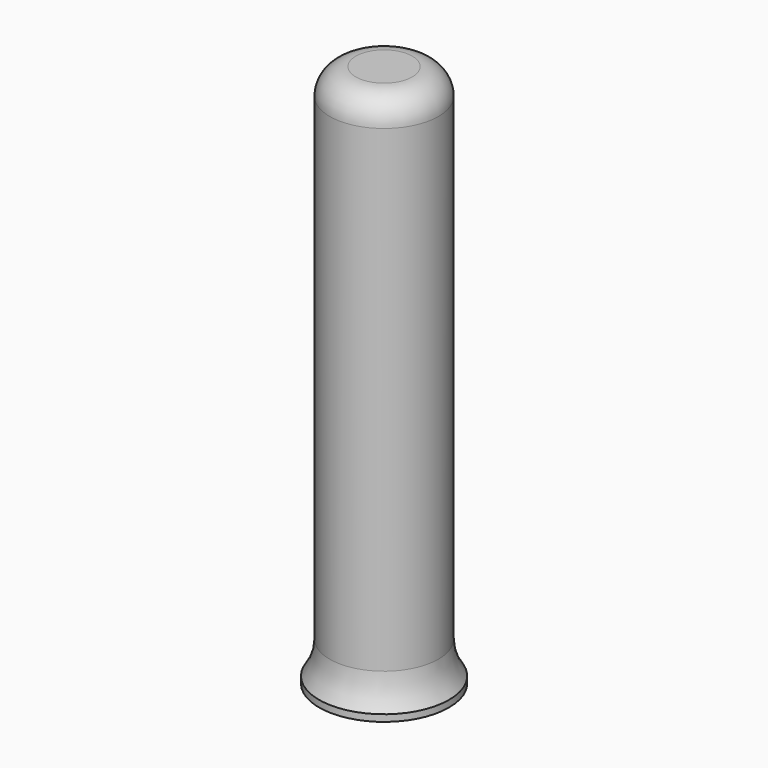
from build123d import *

# Parameters (mm, degrees)
F0_R      = 6.3625068229
F1_DEPTH  = 63.5
F2_R      = 4.7646286231
F3_DEPTH  = 25.146
F4_R      = 7.5920691382
F5_DEPTH  = 0.7874
F6_R      = 4.746247259
F7_DEPTH  = 35.306
F8_R      = 3.0660512242
F10_R     = 4.926173209
F11_DEPTH = 57.658


# Not quite as in the source:
# - a fillet or chamfer that OpenCascade refuses, or shapes differently, is made with other operations: its cross-section is extruded or revolved along the edge and cut away or added


with BuildPart() as f1:
    # F0 (on Top) → F1 (new body)
    with BuildSketch(Plane.XY):
        Circle(F0_R)
    extrude(amount=F1_DEPTH)

    # F2 (on face) → F3 (cut)
    with BuildSketch(Plane(origin=(0, 0, 0), x_dir=(1, 0, 0), z_dir=(0, 0, -1))):
        Circle(F2_R)
    extrude(amount=-F3_DEPTH, mode=Mode.SUBTRACT)

    # F4 (on Top) → F5 (join)
    with BuildSketch(Plane.XY):
        Circle(F4_R)
    extrude(amount=F5_DEPTH)

    # F6 (on face) → F7 (cut)
    with BuildSketch(Plane(origin=(0, 0, 0), x_dir=(1, 0, 0), z_dir=(0, 0, -1))):
        Circle(F6_R)
    extrude(amount=-F7_DEPTH, mode=Mode.SUBTRACT)

    # F8
    f8_edges = [f1.edges().sort_by_distance(p)[0] for p in [
        (-6.362507, 0, 63.5),
    ]]
    fillet(f8_edges, radius=F8_R)

    # F9: fillet of radius 6.4387075708 on 1 edges, made by hand

    # F9_s1 → F9_t2 (revolve)
    with BuildSketch(Plane.XZ):
        with BuildLine():
            ThreePointArc((6.3625068229, 4.5718102432), (6.6776076879, 2.5822384064), (7.5920691382, 0.7874))
            Line((7.5920691382, 0.7874), (6.3625068229, 0.7874))
            Line((6.3625068229, 0.7874), (6.3625068229, 4.5718102432))
        make_face()
    revolve(axis=Axis((0, 0, 0.7874), (0, 0, -1)))

    # F10 (on Top) → F11 (cut)
    with BuildSketch(Plane.XY):
        Circle(F10_R)
    extrude(amount=F11_DEPTH, mode=Mode.SUBTRACT)


solid = f1.part
